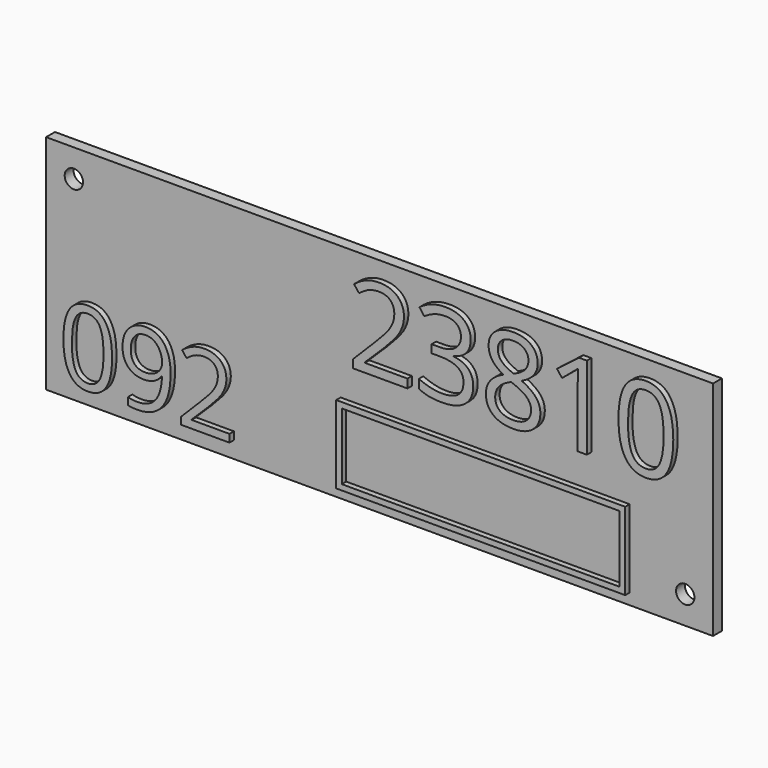
from build123d import *

# Parameters (mm, degrees)
F0_W         = 120
F0_H         = 40
F1_DEPTH     = 2
F3_D         = 3.3
F4_TEXT_SIZE = 20.8786428882
F5_DEPTH     = 1
F6_TEXT_SIZE = 18.5356140827
F7_DEPTH     = 1
F8_W         = 52
F8_H         = 14
F8_W_2       = 49.99999962
F8_H_2       = 11.99999962
F9_DEPTH     = 1


# Not quite as in the source:
# - Text() gives the source's letters only with a copy of the font that has no kerning and outlines rounded to 1/6400 em; it was checked with that copy


with BuildPart() as f1:
    # F0 (on Front) → F1 (new body)
    with BuildSketch(Plane.XZ):
        Rectangle(F0_W, F0_H)
    extrude(amount=F1_DEPTH)

    # F3 (through all)
    with Locations(Plane.XZ.offset(2)):
        with Locations((-55, 15), (55, -15)):
            Hole(F3_D / 2)

    # F4 (on face) → F5 (join)
    with BuildSketch(Plane.XZ.offset(2)):
        with Locations((-5, 2)):
            Text('23810', F4_TEXT_SIZE, font='Open Sans', text_align=(TextAlign.LEFT, TextAlign.BOTTOM))
    extrude(amount=F5_DEPTH)

    # F6 (on face) → F7 (join)
    with BuildSketch(Plane.XZ.offset(2)):
        with Locations((-57, -17)):
            Text('092', F6_TEXT_SIZE, font='Open Sans', text_align=(TextAlign.LEFT, TextAlign.BOTTOM))
    extrude(amount=F7_DEPTH)

    # F8 (on face) → F9 (join)
    with BuildSketch(Plane.XZ.offset(2)):
        with Locations((19, -11)):
            Rectangle(F8_W, F8_H)
        with Locations((19, -11)):
            Rectangle(F8_W_2, F8_H_2, mode=Mode.SUBTRACT)
    extrude(amount=F9_DEPTH)


solid = f1.part
